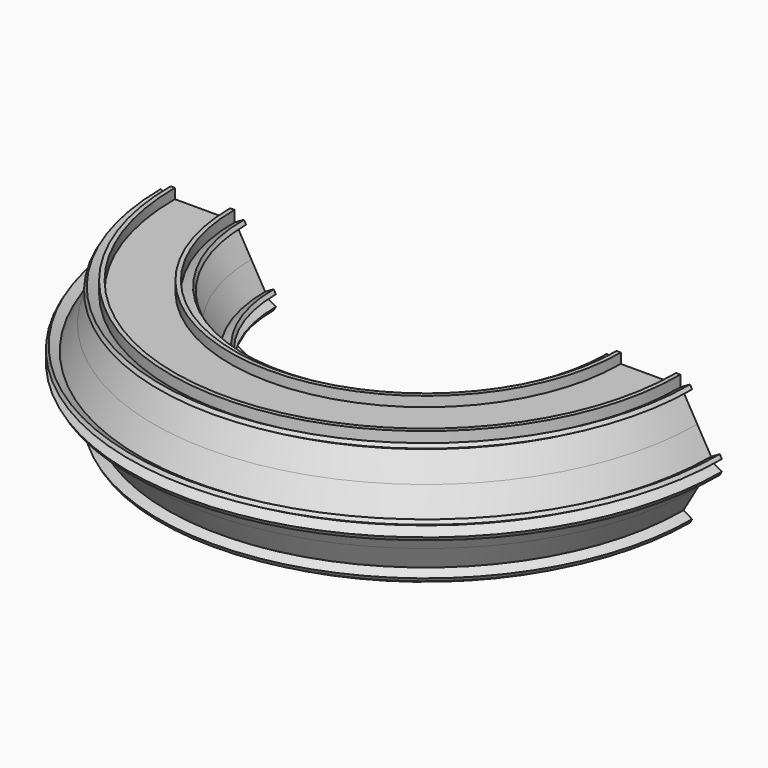
from build123d import *

# Parameters (mm, degrees)
F2_ANGLE = 180


with BuildPart() as f2:
    # F1 (on Front) → F2 (revolve)
    with BuildSketch(Plane.XZ):
        Polygon((-68.0832503253, 1.2704479365), (-65.8827699508, 0), (-68.0832503253, -1.2704479365), (-67.590510429, -2.1238883528), (-65.6038210217, -0.9768590888), (-62.4301136979, -6.4738162454), (-59.2582268861, -11.9676853595), (-61.244893976, -13.1146881387), (-60.7503676631, -13.9712226825), (-58.5499524964, -12.7008123937), (-58.5499524964, -15.2283469215), (-57.5584731996, -15.2283469215), (-57.5584731996, -12.9530243576), (-51.217135042, -12.9530243576), (-44.862665236, -12.9530243576), (-44.862665236, -15.2283469215), (-43.8843175875, -15.2283469215), (-43.8843175875, -12.7008123937), (-41.6742515512, -13.9767946147), (-41.1808964662, -13.1190662144), (-43.1607244284, -11.9802929242), (-39.9959231548, -6.4780897113), (-36.8304619331, -0.9747391376), (-34.850633971, -2.1135124278), (-34.3620503103, -1.2640794445), (-36.5515001331, 0), (-34.3620503103, 1.2640794445), (-34.8630113186, 2.1323707922), (-36.8285001335, 0.9983813071), (-39.9917026714, 6.4810064009), (-43.1661904902, 11.9793805911), (-41.19939244, 13.1149119748), (-41.6910577545, 13.9670915487), (-43.8843175875, 12.7008123937), (-43.8843175875, 15.2525296435), (-44.861279428, 15.2523063589), (-44.861279428, 12.9604106769), (-51.217135042, 12.9604106769), (-57.5630575919, 12.9604106769), (-57.5630575919, 15.2494033683), (-58.5499524964, 15.2491778135), (-58.5499524964, 12.7008123937), (-60.7598529608, 13.9766990217), (-61.2508664965, 13.1247800337), (-59.2498548651, 11.9714734282), (-62.425474964, 6.4711380712), (-65.6057968908, 0.9626589096), (-67.5986398816, 2.1112574229), align=None)
        with BuildLine():
            ThreePointArc((-51.217135042, 12.7008123937), (-42.2363044718, 8.9808305702), (-38.5163226482, 0))
            ThreePointArc((-38.5163226482, 0), (-60.1979656121, -8.9808305702), (-51.217135042, 12.7008123937))
        make_face(mode=Mode.SUBTRACT)
    revolve(axis=Axis((0, 0, 0), (0, 0, 1)), revolution_arc=F2_ANGLE)


solid = f2.part
